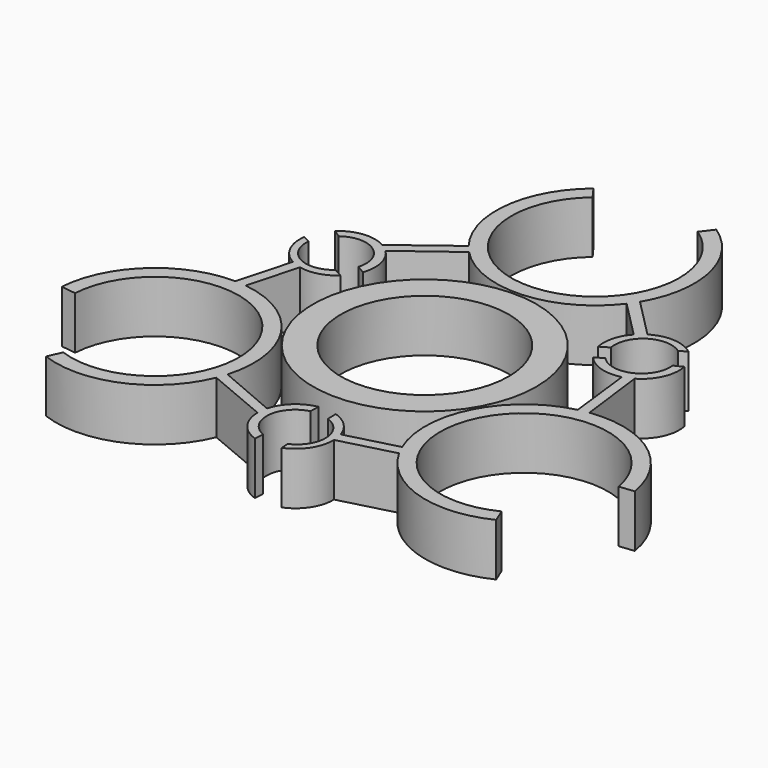
from build123d import *

# Parameters (mm, degrees)
F1_DEPTH = 7
F0_R     = 14.8991210618
F0_R_2   = 11.2


# Not quite as in the source:
# - a feature names something its author has since deleted; it is built from what else it names


with BuildPart() as f1:
    # F0 (on Top) → F1 (new body)
    with BuildSketch(Plane.XY):
        with BuildLine():
            ThreePointArc((6.1727941676, 37.7762980936), (0.6510319855, 17.2498297116), (-7.2157000853, 36.9967355036))
            Line((-7.2157000853, 36.9967355036), (-8.3966559852, 38.6159875526))
            ThreePointArc((-8.3966559852, 38.6159875526), (-13.1168240349, 29.9103945159), (-10.4544622583, 20.3720945463))
            ThreePointArc((-10.4544622583, 20.3720945463), (-10.0184805962, 19.8361235978), (-9.5550524793, 19.3236987275))
            ThreePointArc((-9.5550524793, 19.3236987275), (0.7593543067, 15.2527518823), (10.5378916113, 20.4814997005))
            ThreePointArc((10.5378916113, 20.4814997005), (10.9601407983, 21.0745810082), (11.3490491279, 21.6900402876))
            ThreePointArc((11.3490491279, 21.6900402876), (12.8817645708, 31.3118887778), (7.3962556563, 39.3641168512))
            Line((7.3962556563, 39.3641168512), (6.1727941676, 37.7762980936))
        make_face()
        with BuildLine():
            ThreePointArc((-9.5550524793, 19.3236987275), (-10.0184805962, 19.8361235978), (-10.4544622583, 20.3720945463))
            Line((-10.4544622583, 20.3720945463), (-17.617265947, 14.9386296298))
            ThreePointArc((-17.617265947, 14.9386296298), (-17.0422715879, 14.5599242823), (-16.5243304598, 14.1063019271))
            Line((-16.5243304598, 14.1063019271), (-9.5550524793, 19.3236987275))
        make_face()
        with BuildLine():
            Line((16.5648326928, 16.4198065392), (11.3490491279, 21.6900402876))
            ThreePointArc((11.3490491279, 21.6900402876), (10.9601407983, 21.0745810082), (10.5378916113, 20.4814997005))
            Line((10.5378916113, 20.4814997005), (15.4607146913, 15.5072847985))
            ThreePointArc((15.4607146913, 15.5072847985), (15.9801506346, 16.0030183777), (16.5648326928, 16.4198065392))
        make_face()
        with BuildLine():
            ThreePointArc((22.2866316895, 16.0892831325), (19.4773626659, 17.1483369014), (16.5648326928, 16.4198065392))
            ThreePointArc((16.5648326928, 16.4198065392), (15.9801506346, 16.0030183777), (15.4607146913, 15.5072847985))
            ThreePointArc((15.4607146913, 15.5072847985), (14.3247325692, 13.4259718238), (14.2675578592, 11.0555182525))
            Line((14.2675578592, 11.0555182525), (15.4289464152, 11.7503366329))
            ThreePointArc((15.4289464152, 11.7503366329), (17.1325780757, 15.6513583871), (21.3862302858, 15.4877294253))
            Line((21.3862302858, 15.4877294253), (22.2866316895, 16.0892831325))
        make_face()
        with BuildLine():
            ThreePointArc((-16.5243304598, 14.1063019271), (-17.0422715879, 14.5599242823), (-17.617265947, 14.9386296298))
            ThreePointArc((-17.617265947, 14.9386296298), (-20.6180729349, 15.5614809861), (-23.423944477, 14.3286503897))
            Line((-23.423944477, 14.3286503897), (-22.387528792, 13.6288879439))
            ThreePointArc((-22.387528792, 13.6288879439), (-17.9500491472, 13.7165086278), (-16.4646953344, 9.534089826))
            Line((-16.4646953344, 9.534089826), (-15.3511392531, 8.8629843801))
            ThreePointArc((-15.3511392531, 8.8629843801), (-15.1796922371, 11.6542550315), (-16.5243304598, 14.1063019271))
        make_face()
    extrude(amount=F1_DEPTH)


with BuildPart() as f1b:
    # F0 (on Top) → F1, piece 2 (new body)
    with BuildSketch(Plane.XY):
        Circle(F0_R)
        Circle(F0_R_2, mode=Mode.SUBTRACT)
    extrude(amount=F1_DEPTH)


with BuildPart() as f1c:
    # F0 (on Top) → F1, piece 3 (new body)
    with BuildSketch(Plane.XY):
        with BuildLine():
            ThreePointArc((29.6288367261, -24.2339456083), (14.6132747484, -9.1887250939), (35.6479628458, -12.2493881719))
            Line((35.6479628458, -12.2493881719), (37.6407542054, -12.0362763863))
            ThreePointArc((37.6407542054, -12.0362763863), (32.4615735054, -3.5956944267), (22.8699825346, -1.1322173746))
            ThreePointArc((22.8699825346, -1.1322173746), (22.1878272464, -1.2418030953), (21.5123402327, -1.3869311822))
            ThreePointArc((21.5123402327, -1.3869311822), (12.8295934543, -8.2839960612), (12.4685532426, -19.3668316879))
            ThreePointArc((12.4685532426, -19.3668316879), (12.7710521281, -20.0290508644), (13.1096013342, -20.6735849973))
            ThreePointArc((13.1096013342, -20.6735849973), (20.6760088367, -26.8118797528), (30.3921973626, -26.0874037168))
            Line((30.3921973626, -26.0874037168), (29.6288367261, -24.2339456083))
        make_face()
        with BuildLine():
            ThreePointArc((21.5123402327, -1.3869311822), (22.1878272464, -1.2418030953), (22.8699825346, -1.1322173746))
            Line((22.8699825346, -1.1322173746), (21.7458657307, 7.7876850405))
            ThreePointArc((21.7458657307, 7.7876850405), (21.1304000996, 7.4790779922), (20.4785810523, 7.2573389952))
            Line((20.4785810523, 7.2573389952), (21.5123402327, -1.3869311822))
        make_face()
        with BuildLine():
            ThreePointArc((20.4785810523, 7.2573389952), (21.1304000996, 7.4790779922), (21.7458657307, 7.7876850405))
            ThreePointArc((21.7458657307, 7.7876850405), (23.7856743219, 10.0750344456), (24.1209474779, 13.1214057791))
            Line((24.1209474779, 13.1214057791), (22.9967275808, 12.5737246899))
            ThreePointArc((22.9967275808, 12.5737246899), (20.8538694965, 8.6869442467), (16.4891116585, 9.4917995122))
            Line((16.4891116585, 9.4917995122), (15.3511392531, 8.8629843801))
            ThreePointArc((15.3511392531, 8.8629843801), (17.682727038, 7.3188715832), (20.4785810523, 7.2573389952))
        make_face()
        with BuildLine():
            Line((5.9375532417, -22.555469191), (13.1096013342, -20.6735849973))
            ThreePointArc((13.1096013342, -20.6735849973), (12.7710521281, -20.0290508644), (12.4685532426, -19.3668316879))
            Line((12.4685532426, -19.3668316879), (5.6993452336, -21.1430140826))
            ThreePointArc((5.6993452336, -21.1430140826), (5.868945135, -21.8407255947), (5.9375532417, -22.555469191))
        make_face()
        with BuildLine():
            ThreePointArc((2.7904120767, -27.3454307742), (5.1122140563, -25.4420593181), (5.9375532417, -22.555469191))
            ThreePointArc((5.9375532417, -22.555469191), (5.868945135, -21.8407255947), (5.6993452336, -21.1430140826))
            ThreePointArc((5.6993452336, -21.1430140826), (4.4648663853, -19.1185682192), (2.4405807291, -17.8838266823))
            Line((2.4405807291, -17.8838266823), (2.4616168195, -19.2370278656))
            ThreePointArc((2.4616168195, -19.2370278656), (4.9881849291, -22.6629270394), (2.7196519863, -26.2648834313))
            Line((2.7196519863, -26.2648834313), (2.7904120767, -27.3454307742))
        make_face()
    extrude(amount=F1_DEPTH)


with BuildPart() as f1d:
    # F0 (on Top) → F1, piece 4 (new body)
    with BuildSketch(Plane.XY):
        with BuildLine():
            ThreePointArc((-25.0770437662, 11.2561476417), (-24.5895767222, 8.2937224167), (-22.5023859345, 6.1356626518))
            ThreePointArc((-22.5023859345, 6.1356626518), (-21.8490957696, 5.837707217), (-21.1600599249, 5.6357292841))
            ThreePointArc((-21.1600599249, 5.6357292841), (-18.7895989545, 5.6925963955), (-16.7081385883, 6.8283084297))
            Line((-16.7081385883, 6.8283084297), (-17.8905632347, 7.4866912328))
            ThreePointArc((-17.8905632347, 7.4866912328), (-22.1207630048, 7.0115686523), (-24.1058822721, 10.7771540061))
            Line((-24.1058822721, 10.7771540061), (-25.0770437662, 11.2561476417))
        make_face()
        with BuildLine():
            ThreePointArc((-35.8016308938, -13.5423524853), (-15.264306734, -8.0611046177), (-28.4322627606, -24.7473473317))
            Line((-28.4322627606, -24.7473473317), (-29.2440982202, -26.5797111663))
            ThreePointArc((-29.2440982202, -26.5797111663), (-19.3447494705, -26.3147000891), (-12.4155202763, -19.2398771717))
            ThreePointArc((-12.4155202763, -19.2398771717), (-12.1693466502, -18.5943205025), (-11.9572877534, -17.9367675453))
            ThreePointArc((-11.9572877534, -17.9367675453), (-13.588947761, -6.968755821), (-23.0064448539, -1.1146680126))
            ThreePointArc((-23.0064448539, -1.1146680126), (-23.7311929263, -1.0455301438), (-24.4586504621, -1.0164552902))
            ThreePointArc((-24.4586504621, -1.0164552902), (-33.5577734074, -4.500009025), (-37.7884530188, -13.2767131344))
            Line((-37.7884530188, -13.2767131344), (-35.8016308938, -13.5423524853))
        make_face()
        with BuildLine():
            Line((-22.5023859345, 6.1356626518), (-24.4586504621, -1.0164552902))
            ThreePointArc((-24.4586504621, -1.0164552902), (-23.7311929263, -1.0455301438), (-23.0064448539, -1.1146680126))
            Line((-23.0064448539, -1.1146680126), (-21.1600599249, 5.6357292841))
            ThreePointArc((-21.1600599249, 5.6357292841), (-21.8490957696, 5.837707217), (-22.5023859345, 6.1356626518))
        make_face()
        with BuildLine():
            ThreePointArc((-11.9572877534, -17.9367675453), (-12.1693466502, -18.5943205025), (-12.4155202763, -19.2398771717))
            Line((-12.4155202763, -19.2398771717), (-4.1285997836, -22.7263146703))
            ThreePointArc((-4.1285997836, -22.7263146703), (-4.0881285117, -22.0390022745), (-3.9542505924, -21.3636409223))
            Line((-3.9542505924, -21.3636409223), (-11.9572877534, -17.9367675453))
        make_face()
        with BuildLine():
            ThreePointArc((-3.9542505924, -21.3636409223), (-4.0881285117, -22.0390022745), (-4.1285997836, -22.7263146703))
            ThreePointArc((-4.1285997836, -22.7263146703), (-3.1676013871, -25.6365154318), (-0.6970030009, -27.4500561688))
            Line((-0.6970030009, -27.4500561688), (-0.6091987888, -26.2026126338))
            ThreePointArc((-0.6091987888, -26.2026126338), (-2.9038203493, -22.4034528746), (-0.0244163241, -19.0258893382))
            Line((-0.0244163241, -19.0258893382), (0, -17.7259687602))
            ThreePointArc((0, -17.7259687602), (-2.5030348009, -18.9731266147), (-3.9542505924, -21.3636409223))
        make_face()
    extrude(amount=F1_DEPTH)


solid = Compound([f1.part, f1b.part, f1c.part, f1d.part])
